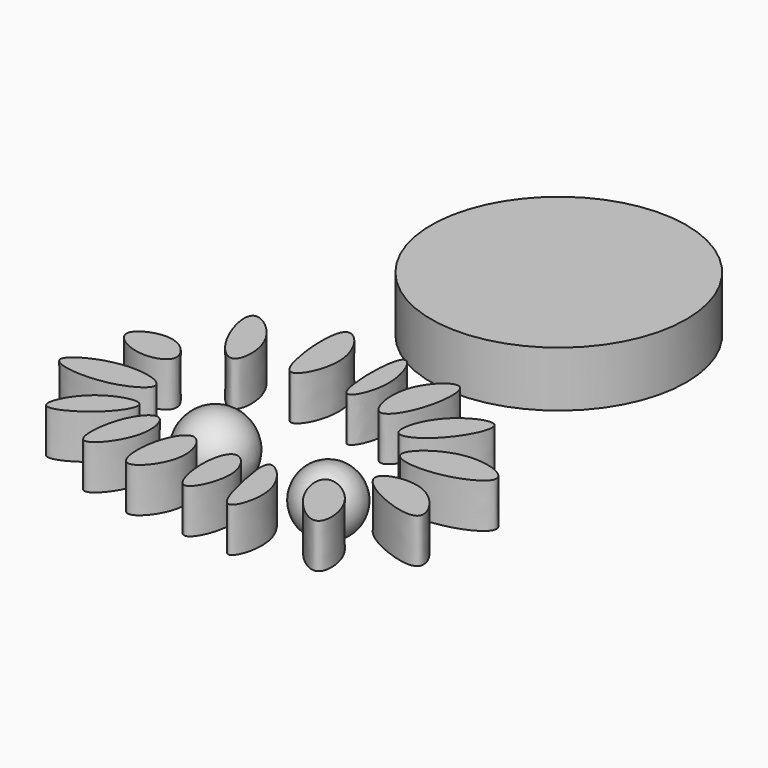
from build123d import *

# Parameters (mm, degrees)
F3_R      = 5.7526414768
F4_DEPTH  = 2.5
F15_DEPTH = 2


# Not quite as in the source:
# - the program builds the solid bodies; features that only make, move or delete a surface that nothing else refers to are left out


with BuildPart() as f4:
    # F3 (on Top) → F4 (new body)
    with BuildSketch(Plane.XY):
        with Locations((0, -20.0255177915)):
            Circle(F3_R)
    extrude(amount=F4_DEPTH)


with BuildPart() as f8:
    # F7 (on Top) → F8 (revolve)
    with BuildSketch(Plane.XY):
        with BuildLine():
            Line((-3.975961823, -32.780982554), (-3.975961823, -36.030061543))
            ThreePointArc((-3.975961823, -36.030061543), (-2.3514223285, -34.4055220485), (-3.975961823, -32.780982554))
        make_face()
    revolve(axis=Axis((-3.975961823, -34.4055220485, 0), (0, 1, 0)))


with BuildPart() as f10:
    # F9 (on Top) → F10 (revolve)
    with BuildSketch(Plane.XY):
        with BuildLine():
            Line((0.6620711647, -35.7757471502), (0.6620711647, -33.2208573818))
            ThreePointArc((0.6620711647, -33.2208573818), (-0.6274149492, -34.498302266), (0.6620711647, -35.7757471502))
        make_face()
    revolve(axis=Axis((0.6620711647, -34.498302266, 0), (0, -1, 0)))


with BuildPart() as f13:
    # F12 (on Top) → F13 (revolve)
    with BuildSketch(Plane.XY):
        with BuildLine():
            Line((1.5284423716, -36.3647043705), (1.5284423716, -33.4796085954))
            ThreePointArc((1.5284423716, -33.4796085954), (0.0756880488, -34.9221564829), (1.5284423716, -36.3647043705))
        make_face()
    revolve(axis=Axis((1.5284423716, -34.9221564829, 0), (0, -1, 0)))


with BuildPart() as f15:
    # F14 (on Top) → F15 (new body)
    with BuildSketch(Plane.XY):
        with BuildLine():
            add(Edge.make_bspline(
                [(-5.4387575947, -31.5687134862), (-5.7361758184, -31.6962112318), (-6.8230946733, -30.5017998629), (-7.4080391918, -27.7899147088), (-5.0094954182, -29.6545878877), (-5.1361401287, -31.4389869206), (-5.4387575947, -31.5687134862)],
                knots=[0, 0, 0, 0, 0.2410933835, 0.4940444095, 0.7546920028, 1, 1, 1, 1], degree=3))
        make_face()
    extrude(amount=F15_DEPTH)


with BuildPart() as f15b:
    # F14 (on Top) → F15, piece 2 (new body)
    with BuildSketch(Plane.XY):
        with BuildLine():
            add(Edge.make_bspline(
                [(-3.771523945, -29.6546053141), (-3.6592855266, -30.4631760253), (-3.203931523, -31.9349610884), (-1.8484101424, -29.0856074499), (-3.8934088824, -26.5156888938), (-3.903219055, -28.7058677054), (-3.771523945, -29.6546053141)],
                knots=[0, 0, 0, 0, 0.2249296539, 0.4841750182, 0.7360784665, 1, 1, 1, 1], degree=3))
        make_face()
    extrude(amount=F15_DEPTH)


with BuildPart() as f15c:
    # F14 (on Top) → F15, piece 3 (new body)
    with BuildSketch(Plane.XY):
        with BuildLine():
            add(Edge.make_bspline(
                [(-7.0701055229, -32.8321307898), (-7.1552436523, -33.1968489636), (-8.393246971, -33.5672151486), (-10.2721897915, -32.3298195992), (-7.9455293959, -31.2727678408), (-6.9818809432, -32.4541907551), (-7.0701055229, -32.8321307898)],
                knots=[0, 0, 0, 0, 0.2394675254, 0.4905165186, 0.7518512338, 1, 1, 1, 1], degree=3))
        make_face()
    extrude(amount=F15_DEPTH)


with BuildPart() as f15d:
    # F14 (on Top) → F15, piece 4 (new body)
    with BuildSketch(Plane.XY):
        with BuildLine():
            add(Edge.make_bspline(
                [(-6.293551065, -34.8794162273), (-6.3415793394, -34.5263834369), (-8.2542822186, -33.9756824599), (-11.2246376935, -35.6343786009), (-7.9201560721, -36.1177993076), (-6.2462698643, -35.2269576375), (-6.293551065, -34.8794162273)],
                knots=[0, 0, 0, 0, 0.2442107033, 0.5019582034, 0.7595879631, 1, 1, 1, 1], degree=3))
        make_face()
    extrude(amount=F15_DEPTH)


with BuildPart() as f15e:
    # F14 (on Top) → F15, piece 5 (new body)
    with BuildSketch(Plane.XY):
        with BuildLine():
            add(Edge.make_bspline(
                [(-5.8589470573, -36.3336652517), (-6.0685415357, -36.0959065752), (-7.8167952944, -36.5444625656), (-8.9686970713, -39.1227807517), (-6.4710876755, -37.8722347214), (-5.6628599287, -36.5561015322), (-5.8589470573, -36.3336652517)],
                knots=[0, 0, 0, 0, 0.2520910184, 0.5046640867, 0.7641550278, 1, 1, 1, 1], degree=3))
        make_face()
    extrude(amount=F15_DEPTH)


with BuildPart() as f15f:
    # F14 (on Top) → F15, piece 6 (new body)
    with BuildSketch(Plane.XY):
        with BuildLine():
            add(Edge.make_bspline(
                [(-4.7046658583, -36.7014855146), (-4.9900118712, -36.6079710076), (-5.8750873735, -37.5914329093), (-6.02642237, -40.6757504606), (-4.0289800412, -38.313505601), (-4.3988223274, -36.8017175338), (-4.7046658583, -36.7014855146)],
                knots=[0, 0, 0, 0, 0.2232617478, 0.4953587973, 0.7607004893, 1, 1, 1, 1], degree=3))
        make_face()
    extrude(amount=F15_DEPTH)


with BuildPart() as f15g:
    # F14 (on Top) → F15, piece 7 (new body)
    with BuildSketch(Plane.XY):
        with BuildLine():
            add(Edge.make_bspline(
                [(-2.8190067969, -37.0910093188), (-3.171340113, -37.0518845994), (-3.8911802065, -38.3517376539), (-3.6144463033, -40.9551724075), (-1.7041183969, -38.6810398837), (-2.4573028574, -37.1311745956), (-2.8190067969, -37.0910093188)],
                knots=[0, 0, 0, 0, 0.2392295055, 0.4913719997, 0.7544079692, 1, 1, 1, 1], degree=3))
        make_face()
    extrude(amount=F15_DEPTH)


with BuildPart() as f15h:
    # F14 (on Top) → F15, piece 8 (new body)
    with BuildSketch(Plane.XY):
        with BuildLine():
            add(Edge.make_bspline(
                [(-0.8024710696, -37.2487381101), (-1.1116109992, -37.2928047097), (-1.4738461334, -38.5645485256), (-0.7950255017, -41.1156516149), (0.4544305492, -38.3075757851), (-0.4984355796, -37.2053991269), (-0.8024710696, -37.2487381101)],
                knots=[0, 0, 0, 0, 0.2358135977, 0.4921981834, 0.7680800962, 1, 1, 1, 1], degree=3))
        make_face()
    extrude(amount=F15_DEPTH)


with BuildPart() as f15i:
    # F14 (on Top) → F15, piece 9 (new body)
    with BuildSketch(Plane.XY):
        with BuildLine():
            add(Edge.make_bspline(
                [(0.6435168907, -37.0701104403), (0.4186035253, -37.1100855391), (0.5482737206, -38.3503739671), (1.3269723466, -41.3875550584), (2.3064110082, -38.4050757448), (0.9191361748, -37.0211230975), (0.6435168907, -37.0701104403)],
                knots=[0, 0, 0, 0, 0.2104665868, 0.4870432031, 0.7420844693, 1, 1, 1, 1], degree=3))
        make_face()
    extrude(amount=F15_DEPTH)


with BuildPart() as f15j:
    # F14 (on Top) → F15, piece 10 (new body)
    with BuildSketch(Plane.XY):
        with BuildLine():
            add(Edge.make_bspline(
                [(2.8969747946, -36.7065966129), (2.5987607902, -36.8574285168), (2.7195080443, -38.2609289942), (4.9646642717, -40.1991367345), (4.8272586066, -37.4512286214), (3.2406687316, -36.5327616819), (2.8969747946, -36.7065966129)],
                knots=[0, 0, 0, 0, 0.2243097554, 0.4951585463, 0.7414812791, 1, 1, 1, 1], degree=3))
        make_face()
    extrude(amount=F15_DEPTH)


with BuildPart() as f15k:
    # F14 (on Top) → F15, piece 11 (new body)
    with BuildSketch(Plane.XY):
        with BuildLine():
            add(Edge.make_bspline(
                [(4.14360594, -35.4162752628), (4.0096445879, -35.7299275447), (5.0884361999, -36.6428593789), (7.9610907546, -37.4392167615), (6.2139331116, -34.6259951538), (4.2935074406, -35.0653012921), (4.14360594, -35.4162752628)],
                knots=[0, 0, 0, 0, 0.2249450914, 0.4867710464, 0.748288546, 1, 1, 1, 1], degree=3))
        make_face()
    extrude(amount=F15_DEPTH)


with BuildPart() as f15l:
    # F14 (on Top) → F15, piece 12 (new body)
    with BuildSketch(Plane.XY):
        with BuildLine():
            add(Edge.make_bspline(
                [(3.7330486812, -33.5862785578), (3.8161754189, -33.9857823985), (5.7916836014, -34.2121096373), (8.466159551, -32.8516766833), (5.4070031907, -31.7342289603), (3.6465619741, -33.1706268365), (3.7330486812, -33.5862785578)],
                knots=[0, 0, 0, 0, 0.2460458568, 0.4934871631, 0.7440090094, 1, 1, 1, 1], degree=3))
        make_face()
    extrude(amount=F15_DEPTH)


with BuildPart() as f15m:
    # F14 (on Top) → F15, piece 13 (new body)
    with BuildSketch(Plane.XY):
        with BuildLine():
            add(Edge.make_bspline(
                [(2.6498879306, -32.3671326041), (2.8839957399, -32.5925284124), (4.2580963943, -31.8855396899), (5.6105522442, -29.1169465394), (2.8549987909, -30.2706837941), (2.3903344443, -32.1172380448), (2.6498879306, -32.3671326041)],
                knots=[0, 0, 0, 0, 0.229003799, 0.4952324342, 0.7461052898, 1, 1, 1, 1], degree=3))
        make_face()
    extrude(amount=F15_DEPTH)


with BuildPart() as f15n:
    # F14 (on Top) → F15, piece 14 (new body)
    with BuildSketch(Plane.XY):
        with BuildLine():
            add(Edge.make_bspline(
                [(1.1442401446, -31.5370708704), (1.4582674622, -31.645640201), (2.3204959252, -30.3939228223), (2.5195077461, -27.4211974137), (0.296422183, -29.3957551255), (0.7824559149, -31.4119904413), (1.1442401446, -31.5370708704)],
                knots=[0, 0, 0, 0, 0.2269981488, 0.4913743883, 0.7384802346, 1, 1, 1, 1], degree=3))
        make_face()
    extrude(amount=F15_DEPTH)


with BuildPart() as f15o:
    # F14 (on Top) → F15, piece 15 (new body)
    with BuildSketch(Plane.XY):
        with BuildLine():
            add(Edge.make_bspline(
                [(-0.6937938742, -31.1245899647), (-0.4361242639, -31.3808804429), (0.4524688405, -29.6238807647), (-1.0923689255, -26.3428987985), (-1.0530062388, -30.7673002225), (-0.6937938742, -31.1245899647)],
                knots=[0, 0, 0, 0, 0.289371327, 0.5965928677, 1, 1, 1, 1], degree=3))
        make_face()
    extrude(amount=F15_DEPTH)


solid = Compound([f4.part, f8.part, f13.part, f15.part, f15b.part, f15c.part, f15d.part, f15e.part, f15f.part, f15g.part, f15h.part, f15i.part, f15j.part, f15k.part, f15l.part, f15m.part, f15n.part, f15o.part])
